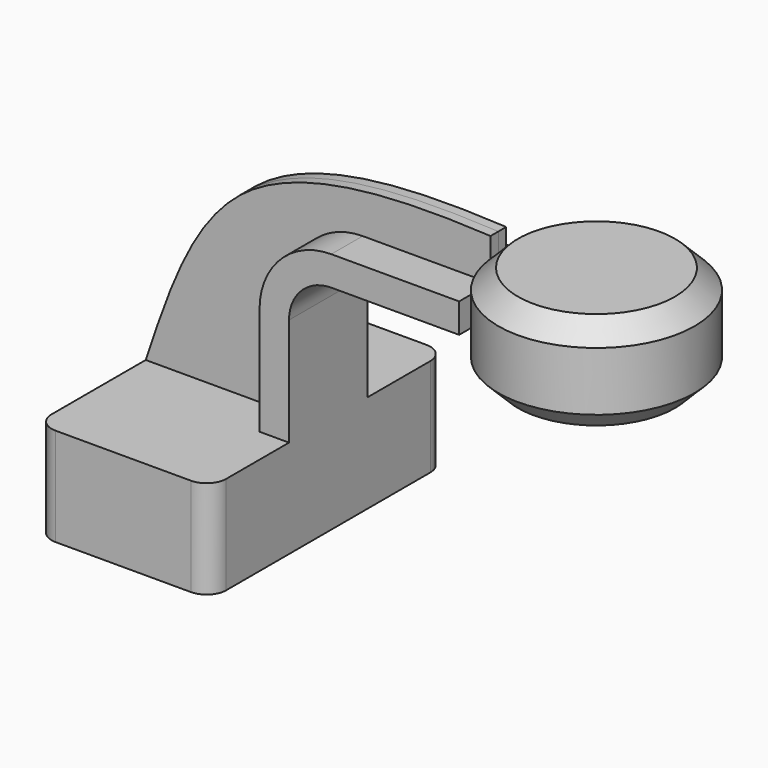
from build123d import *

# Parameters (mm, degrees)
F1_DEPTH    = 38.1
F2_DEPTH    = 2.54
F0_W        = 25.4
F0_H        = 25.4
F4_DEPTH    = 12.7
F5_R        = 5.08
F6_T2_ANGLE = 180
F6_T4_ANGLE = 180


# Not quite as in the source:
# - a fillet or chamfer that OpenCascade refuses, or shapes differently, is made with other operations: its cross-section is extruded or revolved along the edge and cut away or added


with BuildPart() as f1:
    # F0 (on Front) → F1 (new body, symmetric)
    with BuildSketch(Plane.XZ):
        Polygon((-44.2866310477, 25.4), (-44.2866310477, 0), (0.9434421729, 0), (0.9434421729, 25.4), (-6.6829477437, 25.4), align=None)
    extrude(amount=F1_DEPTH, both=True)

    # F0 (on Front) → F2 (join, symmetric)
    with BuildSketch(Plane.XZ):
        with BuildLine():
            add(Edge.make_bspline(
                [(44.9969768524, 82.6969615459), (20.8074855996, 83.9490606701), (-25.6210994511, 82.0372772331), (-38.1906192957, 43.6191001085), (-44.2866310477, 25.4)],
                knots=[0, 0, 0, 0, 0.5240773197, 1, 1, 1, 1], degree=3))
            Line((-44.2866310477, 25.4), (-6.6829477437, 25.4))
            Line((-6.6829477437, 25.4), (-6.6829477437, 53.3393811594))
            ThreePointArc((-6.6829477437, 53.3393811594), (-1.2412562476, 66.4767865715), (11.8961491644, 71.9184780675))
            Line((11.8961491644, 71.9184780675), (44.9969768524, 71.9184780675))
            Line((44.9969768524, 71.9184780675), (44.9969768524, 82.6969615459))
        make_face()
    extrude(amount=F2_DEPTH, both=True)

    # F0 (on Front) → F3 (revolve)
    with BuildSketch(Plane.XZ):
        with Locations((83.0969768524, 69.9969615459)):
            Rectangle(F0_W, F0_H)
    revolve(axis=Axis((70.3969768524, 0, 69.9969615459), (0, 0, 1)))

    # F0 (on Front) → F4 (join, symmetric)
    with BuildSketch(Plane.XZ):
        with BuildLine():
            Line((-6.6829477437, 25.4), (0.9434421729, 25.4))
            Line((0.9434421729, 25.4), (0.9434421729, 53.3393811594))
            ThreePointArc((0.9434421729, 53.3393811594), (4.1514157783, 61.0841145455), (11.8961491644, 64.292088151))
            Line((11.8961491644, 64.292088151), (44.9969768524, 64.292088151))
            Line((44.9969768524, 64.292088151), (44.9969768524, 71.9184780675))
            Line((44.9969768524, 71.9184780675), (11.8961491644, 71.9184780675))
            ThreePointArc((11.8961491644, 71.9184780675), (-1.2412562476, 66.4767865715), (-6.6829477437, 53.3393811594))
            Line((-6.6829477437, 53.3393811594), (-6.6829477437, 25.4))
        make_face()
    extrude(amount=F4_DEPTH, both=True)

    # F5
    f5_edges = [f1.edges().sort_by_distance(p)[0] for p in [
        (-44.286631, -38.1, 12.7),
        (0.943442, -38.1, 12.7),
        (0.943442, 38.1, 12.7),
        (-44.286631, 38.1, 12.7),
    ]]
    fillet(f5_edges, radius=F5_R)

    # F6: chamfer of 5.08 on 3 edges, made by hand

    # F6_s1 → F6_t2 (revolve, cut)
    with BuildSketch(Plane.XZ):
        Polygon((95.7969768524, 77.6169615459), (90.7169768524, 82.6969615459), (95.7969768524, 82.6969615459), align=None)
    revolve(axis=Axis((70.3969768524, 0, 82.6969615459), (0, 0, 1)), revolution_arc=F6_T2_ANGLE, mode=Mode.SUBTRACT)

    # F6_s3 → F6_t4 (revolve, cut)
    with BuildSketch(Plane.XZ):
        Polygon((44.9969768524, 77.6169615459), (50.0769768524, 82.6969615459), (44.9969768524, 82.6969615459), align=None)
    revolve(axis=Axis((70.3969768524, 0, 82.6969615459), (0, 0, 1)), revolution_arc=F6_T4_ANGLE, mode=Mode.SUBTRACT)

    # F6_s5 → F6_t6 (revolve, cut)
    with BuildSketch(Plane.XZ):
        Polygon((95.7969768524, 62.3769615459), (90.7169768524, 57.2969615459), (95.7969768524, 57.2969615459), align=None)
    revolve(axis=Axis((70.3969768524, 0, 57.2969615459), (0, 0, 1)), mode=Mode.SUBTRACT)


solid = f1.part
